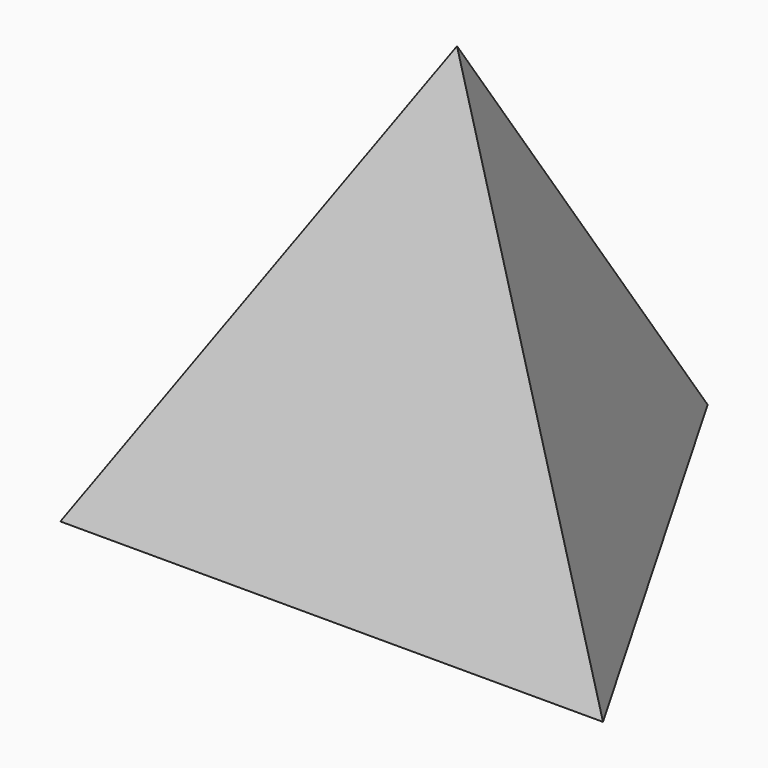
from build123d import *

# Parameters (mm, degrees)
F2_DEPTH = 1000
F2_TAPER = 19.471


with BuildPart() as f2:
    # F0 (on Top) → F2 (new body)
    with BuildSketch(Plane.XY):
        Polygon((0, 0), (0, 115.470054), (-100, -57.735027), align=None)
        Polygon((100, -57.735027), (0, 115.470054), (0, 0), align=None)
        Polygon((-100, -57.735027), (100, -57.735027), (0, 0), align=None)
    extrude(amount=F2_DEPTH, taper=F2_TAPER)


solid = f2.part
